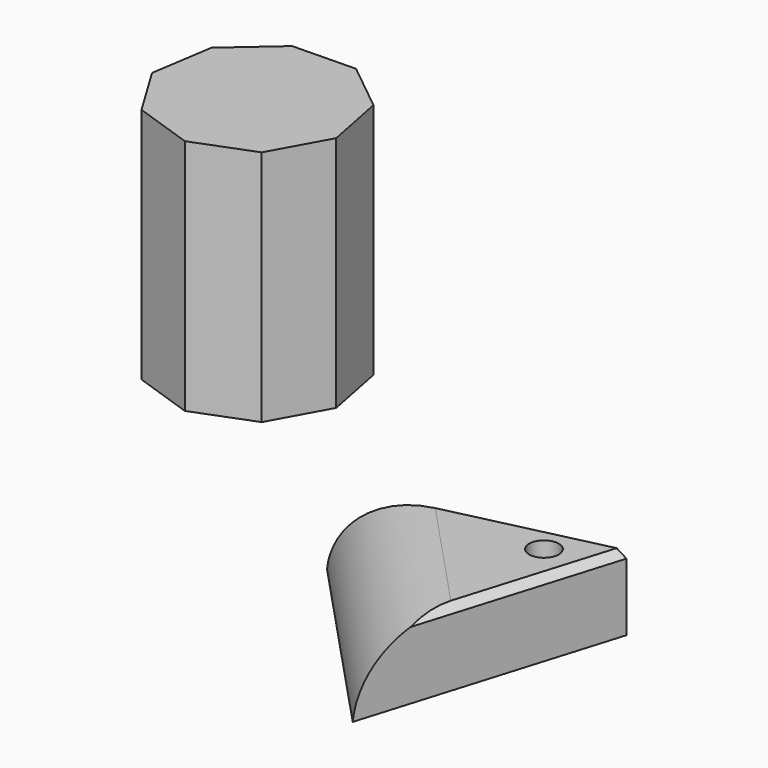
from build123d import *

# Parameters (mm, degrees)
F1_DEPTH    = 51
F2_T1_DEPTH = 202.5458455168
F3_T1_DEPTH = 447.7658767431
F4_R        = 10.0685716687
F5_DEPTH    = 111
F7_DEPTH    = 162


# Not quite as in the source:
# - a fillet or chamfer that OpenCascade refuses, or shapes differently, is made with other operations: its cross-section is extruded or revolved along the edge and cut away or added


with BuildPart() as f1:
    # F0 (on Top) → F1 (new body)
    with BuildSketch(Plane.XY):
        Polygon((-66.8284512856, -91.2451116348), (-15.4423944853, 77.9529200846), (-187.6652166247, 37.8555348143), align=None)
    extrude(amount=F1_DEPTH)

    # F2: chamfer of 5 on 1 edges, made by hand

    # F2_s2 → F2_t1 (cut)
    with BuildSketch(Plane(origin=(-34.7514003583, -114.42536957, 0), x_dir=(0, 0, 1), z_dir=(0.2905974261, 0.9568454086, 0))):
        Polygon((46, -37.428902193), (51, -42.428902193), (51, -37.428902193), align=None)
    extrude(amount=F2_T1_DEPTH, mode=Mode.SUBTRACT)

    # F3: fillet of radius 55.5269119346 on 1 edges, made by hand

    # F3_s2 → F3_t1 (cut)
    with BuildSketch(Plane(origin=(-201.066415005, 214.8171054023, 0), x_dir=(0, 0, 1), z_dir=(0.6833537183, -0.7300874576, 0))):
        with BuildLine():
            ThreePointArc((0, 111.1433004041), (36.3056938439, 93.4301560684), (51, 55.8012276445))
            Line((51, 55.8012276445), (51, 111.1433004041))
            Line((51, 111.1433004041), (0, 111.1433004041))
        make_face()
    extrude(amount=F3_T1_DEPTH, mode=Mode.SUBTRACT)

    # F4 (on face) → F5 (cut)
    with BuildSketch(Plane.XY.offset(51)):
        with Locations((-50.6426393986, 51.6071207821)):
            Circle(F4_R)
    extrude(amount=-F5_DEPTH, mode=Mode.SUBTRACT)


with BuildPart() as f7:
    # F6 (on Top) → F7 (new body)
    with BuildSketch(Plane.XY):
        Polygon((-360.7626209722, 133.0184859606), (-320.7055081859, 148.5207455781), (-299.9846399328, 186.1443811928), (-308.2955407554, 228.2848755603), (-341.7494477934, 255.2242230267), (-384.6929061449, 254.357203515), (-417.0321943839, 226.0895050905), (-423.6354001323, 183.6478980066), (-401.4128100338, 146.8912819037), align=None)
    extrude(amount=F7_DEPTH)


solid = Compound([f1.part, f7.part])
